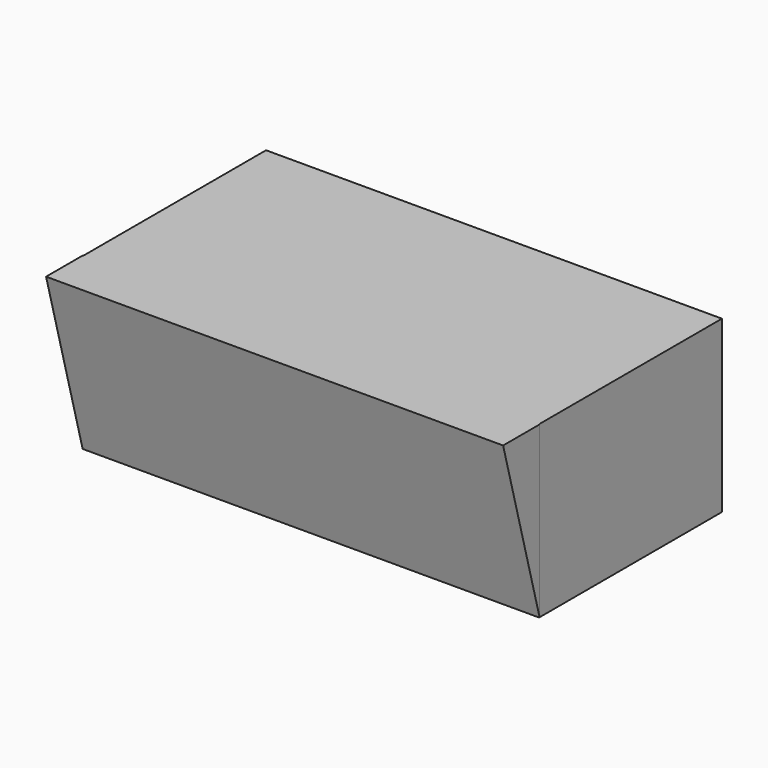
from build123d import *

# Parameters (mm, degrees)
F0_W        = 79.8
F0_H        = 29.8
F1_DEPTH    = 20
F3_DEPTH    = 40
F4_T        = 2
F4_T3_DEPTH = 33.8


# Not quite as in the source:
# - a shell that OpenCascade refuses in one call is made with other operations: the cavity is built on its own and cut out


with BuildPart() as f1:
    # F0 (on Front) → F1 (new body, symmetric)
    with BuildSketch(Plane.XZ):
        Rectangle(F0_W, F0_H)
    extrude(amount=F1_DEPTH, both=True)

    # F2 (on Right) → F3 (join, symmetric)
    with BuildSketch(Plane.YZ):
        Polygon((-28, 14.9), (-20, -14.9), (-20, 14.9), align=None)
    extrude(amount=F3_DEPTH, both=True)

    # F4: shell of thickness 2, made by hand


with BuildPart() as f4_core1:
    # F4_t2: copy of F1
    add(f1.part)

    # the walls: a layer under each face that stays
    f4_faces = [f4_core1.faces().sort_by_distance(p)[0] for p in [
        (0, -24, 0),
        (-40, -24, 9.9333333333),
        (-39.95, -20, 0),
        (0, 0, -14.9),
        (39.95, -20, 0),
        (40, -24, 9.9333333333),
        (0, -4, 14.9),
        (-39.9, 0, 0),
        (39.9, 0, 0),
    ]]
    thicken(f4_faces, amount=-F4_T, mode=Mode.SUBTRACT)

    # F4_s4 → F4_t3 (cut)
    with BuildSketch(Plane.XY.offset(-16.9)):
        Polygon((-39.92, -19.98), (-39.9, -22), (-37.9, -22), (-37.9, -20), align=None)
        Polygon((39.92, -19.98), (39.9, -22), (37.9, -22), (37.9, -20), align=None)
    extrude(amount=F4_T3_DEPTH, mode=Mode.SUBTRACT)


with BuildPart() as f1_1:
    add(f1.part)

    # what is left inside the walls is the cavity
    f4_cavity = [f4_core1.part.solids().sort_by_distance(p)[0] for p in [
        (-12.666667, -2.696136, 12.88),
    ]]
    add(f4_cavity, mode=Mode.SUBTRACT)


solid = f1_1.part
